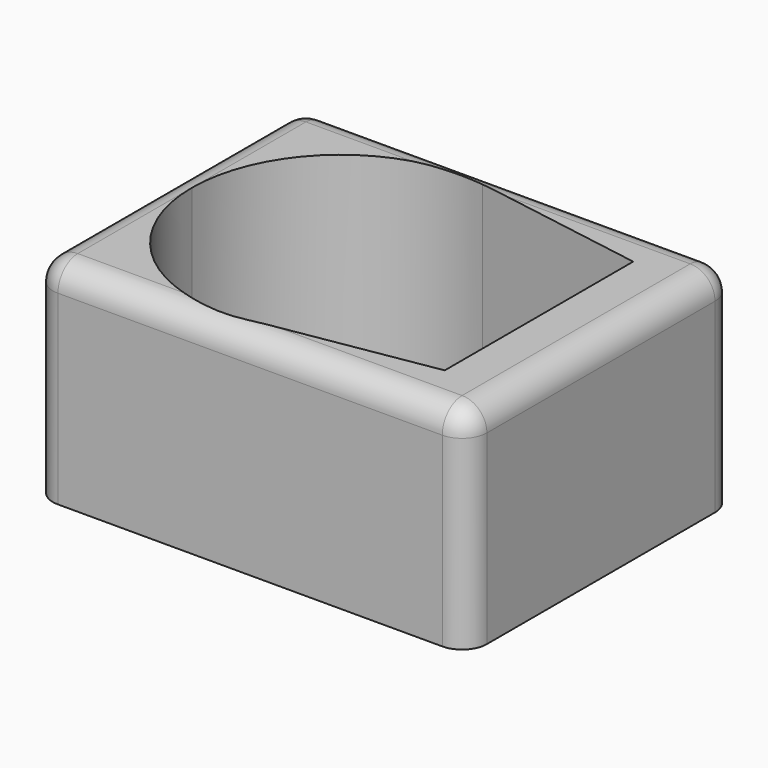
from build123d import *

# Parameters (mm, degrees)
F0_W         = 35
F0_H         = 27
F1_DEPTH     = 15
F2_DEPTH     = 2
F3_T1_DEPTH  = 20
F3_T3_DEPTH  = 23
F3_T5_DEPTH  = 31
F3_S9_W      = 2
F3_S9_H      = 2
F3_T10_DEPTH = 2
F3_S15_W     = 2
F3_S15_H     = 2
F3_T16_DEPTH = 2
F3_S21_W     = 2
F3_S21_H     = 2
F3_T22_DEPTH = 2
F3_S27_W     = 2
F3_S27_H     = 2
F3_T28_DEPTH = 2


# Not quite as in the source:
# - a fillet or chamfer that OpenCascade refuses, or shapes differently, is made with other operations: its cross-section is extruded or revolved along the edge and cut away or added


with BuildPart() as f1:
    # F0 (on Top) → F1 (new body)
    with BuildSketch(Plane.XY):
        with Locations((-13.2022674233, 7.6325895488)):
            Rectangle(F0_W, F0_H)
        with BuildLine():
            Line((-14.73041686, 19.4694728107), (-0.7022674233, 17.1325895488))
            Line((-0.7022674233, 17.1325895488), (-0.7022674233, 7.6325895488))
            Line((-0.7022674233, 7.6325895488), (-0.7022674233, -1.8674104512))
            Line((-0.7022674233, -1.8674104512), (-14.73041686, -4.2042937131))
            ThreePointArc((-14.73041686, -4.2042937131), (-24.4591286842, -1.5233431387), (-28.7022674233, 7.6325895488))
            ThreePointArc((-28.7022674233, 7.6325895488), (-24.4591286842, 16.7885222364), (-14.73041686, 19.4694728107))
        make_face(mode=Mode.SUBTRACT)
    extrude(amount=F1_DEPTH)

    # F0 (on Top) → F2 (join)
    with BuildSketch(Plane.XY):
        with Locations((-13.2022674233, 7.6325895488)):
            Rectangle(F0_W, F0_H)
        with BuildLine():
            Line((-14.73041686, 19.4694728107), (-0.7022674233, 17.1325895488))
            Line((-0.7022674233, 17.1325895488), (-0.7022674233, 7.6325895488))
            Line((-0.7022674233, 7.6325895488), (-0.7022674233, -1.8674104512))
            Line((-0.7022674233, -1.8674104512), (-14.73041686, -4.2042937131))
            ThreePointArc((-14.73041686, -4.2042937131), (-24.4591286842, -1.5233431387), (-28.7022674233, 7.6325895488))
            ThreePointArc((-28.7022674233, 7.6325895488), (-24.4591286842, 16.7885222364), (-14.73041686, 19.4694728107))
        make_face(mode=Mode.SUBTRACT)
        with BuildLine():
            ThreePointArc((-14.73041686, -4.2042937131), (-7.5463347357, -0.1242717121), (-4.7022674233, 7.6325895488))
            Line((-4.7022674233, 7.6325895488), (-28.7022674233, 7.6325895488))
            ThreePointArc((-28.7022674233, 7.6325895488), (-24.4591286842, -1.5233431387), (-14.73041686, -4.2042937131))
        make_face()
        with BuildLine():
            ThreePointArc((-4.7022674233, 7.6325895488), (-7.5463347357, 15.3894508097), (-14.73041686, 19.4694728107))
            ThreePointArc((-14.73041686, 19.4694728107), (-24.4591286842, 16.7885222364), (-28.7022674233, 7.6325895488))
            Line((-28.7022674233, 7.6325895488), (-4.7022674233, 7.6325895488))
        make_face()
        with BuildLine():
            Line((-0.7022674233, 7.6325895488), (-0.7022674233, 17.1325895488))
            Line((-0.7022674233, 17.1325895488), (-14.73041686, 19.4694728107))
            ThreePointArc((-14.73041686, 19.4694728107), (-7.5463347357, 15.3894508097), (-4.7022674233, 7.6325895488))
            Line((-4.7022674233, 7.6325895488), (-0.7022674233, 7.6325895488))
        make_face()
        with BuildLine():
            Line((-0.7022674233, -1.8674104512), (-0.7022674233, 7.6325895488))
            Line((-0.7022674233, 7.6325895488), (-4.7022674233, 7.6325895488))
            ThreePointArc((-4.7022674233, 7.6325895488), (-7.5463347357, -0.1242717121), (-14.73041686, -4.2042937131))
            Line((-14.73041686, -4.2042937131), (-0.7022674233, -1.8674104512))
        make_face()
    extrude(amount=-F2_DEPTH)

    # F3: fillet of radius 2 on 8 edges, made by hand

    # F3_s2 → F3_t1 (cut)
    with BuildSketch(Plane.XY.offset(-7)):
        with BuildLine():
            ThreePointArc((-30.7022674233, -3.8674104512), (-30.1164809856, -5.2816240135), (-28.7022674233, -5.8674104512))
            Line((-28.7022674233, -5.8674104512), (-30.7022674233, -5.8674104512))
            Line((-30.7022674233, -5.8674104512), (-30.7022674233, -3.8674104512))
        make_face()
        with BuildLine():
            ThreePointArc((-30.7022674233, 19.1325895488), (-30.1164809856, 20.5468031112), (-28.7022674233, 21.1325895488))
            Line((-28.7022674233, 21.1325895488), (-30.7022674233, 21.1325895488))
            Line((-30.7022674233, 21.1325895488), (-30.7022674233, 19.1325895488))
        make_face()
        with BuildLine():
            ThreePointArc((4.2977325767, -3.8674104512), (3.7119461391, -5.2816240135), (2.2977325767, -5.8674104512))
            Line((2.2977325767, -5.8674104512), (4.2977325767, -5.8674104512))
            Line((4.2977325767, -5.8674104512), (4.2977325767, -3.8674104512))
        make_face()
        with BuildLine():
            ThreePointArc((4.2977325767, 19.1325895488), (3.7119461391, 20.5468031112), (2.2977325767, 21.1325895488))
            Line((2.2977325767, 21.1325895488), (4.2977325767, 21.1325895488))
            Line((4.2977325767, 21.1325895488), (4.2977325767, 19.1325895488))
        make_face()
    extrude(amount=F3_T1_DEPTH, mode=Mode.SUBTRACT)

    # F3_s4 → F3_t3 (cut)
    with BuildSketch(Plane.XZ.offset(-19.1325895488)):
        with BuildLine():
            ThreePointArc((-30.7022674233, 13), (-30.1164809856, 14.4142135624), (-28.7022674233, 15))
            Line((-28.7022674233, 15), (-30.7022674233, 15))
            Line((-30.7022674233, 15), (-30.7022674233, 13))
        make_face()
        with BuildLine():
            ThreePointArc((4.2977325767, 13), (3.7119461391, 14.4142135624), (2.2977325767, 15))
            Line((2.2977325767, 15), (4.2977325767, 15))
            Line((4.2977325767, 15), (4.2977325767, 13))
        make_face()
    extrude(amount=F3_T3_DEPTH, mode=Mode.SUBTRACT)

    # F3_s6 → F3_t5 (cut)
    with BuildSketch(Plane.YZ.offset(-28.7022674233)):
        with BuildLine():
            ThreePointArc((21.1325895488, 13), (20.5468031112, 14.4142135624), (19.1325895488, 15))
            Line((19.1325895488, 15), (21.1325895488, 15))
            Line((21.1325895488, 15), (21.1325895488, 13))
        make_face()
        with BuildLine():
            ThreePointArc((-3.8674104512, 15), (-5.2816240135, 14.4142135624), (-5.8674104512, 13))
            Line((-5.8674104512, 13), (-5.8674104512, 15))
            Line((-5.8674104512, 15), (-3.8674104512, 15))
        make_face()
    extrude(amount=F3_T5_DEPTH, mode=Mode.SUBTRACT)


with BuildPart() as f3_tool8:
    # F3_s9 → F3_t10 (new body)
    with BuildSketch(Plane.YZ.offset(-28.7022674233)):
        with Locations((-4.8674104512, 14)):
            Rectangle(F3_S9_W, F3_S9_H)
    extrude(amount=-F3_T10_DEPTH)

    # F3_s11 → F3_t12 (revolve, cut)
    with BuildSketch(Plane(origin=(-28.7022674233, -3.8674104512, 13), x_dir=(0, 0.7071067812, -0.7071067812), z_dir=(0, 0.7071067812, 0.7071067812))):
        with BuildLine():
            ThreePointArc((0, -2), (2, 0), (0, 2))
            Line((0, 2), (0, -2))
        make_face()
    revolve(axis=Axis((-28.7022674233, -3.8674104512, 13), (-1, 0, 0)), mode=Mode.SUBTRACT)


with BuildPart() as f1_1:
    add(f1.part)

    # F3_t7: cut F3_tool8
    add(f3_tool8.part, mode=Mode.SUBTRACT)


with BuildPart() as f3_tool14:
    # F3_s15 → F3_t16 (new body)
    with BuildSketch(Plane.YZ.offset(-28.7022674233)):
        with Locations((20.1325895488, 14)):
            Rectangle(F3_S15_W, F3_S15_H)
    extrude(amount=-F3_T16_DEPTH)

    # F3_s17 → F3_t18 (revolve, cut)
    with BuildSketch(Plane(origin=(-28.7022674233, 19.1325895488, 13), x_dir=(0, -0.7071067812, -0.7071067812), z_dir=(0, 0.7071067812, -0.7071067812))):
        with BuildLine():
            ThreePointArc((0, -2), (2, 0), (0, 2))
            Line((0, 2), (0, -2))
        make_face()
    revolve(axis=Axis((-28.7022674233, 19.1325895488, 13), (-1, 0, 0)), mode=Mode.SUBTRACT)


with BuildPart() as f1_2:
    add(f1_1.part)

    # F3_t13: cut F3_tool14
    add(f3_tool14.part, mode=Mode.SUBTRACT)


with BuildPart() as f3_tool20:
    # F3_s21 → F3_t22 (new body)
    with BuildSketch(Plane.YZ.offset(2.2977325767)):
        with Locations((20.1325895488, 14)):
            Rectangle(F3_S21_W, F3_S21_H)
    extrude(amount=F3_T22_DEPTH)

    # F3_s23 → F3_t24 (revolve, cut)
    with BuildSketch(Plane(origin=(2.2977325767, 19.1325895488, 13), x_dir=(0, -0.7071067812, -0.7071067812), z_dir=(0, -0.7071067812, 0.7071067812))):
        with BuildLine():
            ThreePointArc((0, -2), (2, 0), (0, 2))
            Line((0, 2), (0, -2))
        make_face()
    revolve(axis=Axis((2.2977325767, 19.1325895488, 13), (1, 0, 0)), mode=Mode.SUBTRACT)


with BuildPart() as f1_3:
    add(f1_2.part)

    # F3_t19: cut F3_tool20
    add(f3_tool20.part, mode=Mode.SUBTRACT)


with BuildPart() as f3_tool26:
    # F3_s27 → F3_t28 (new body)
    with BuildSketch(Plane.YZ.offset(2.2977325767)):
        with Locations((-4.8674104512, 14)):
            Rectangle(F3_S27_W, F3_S27_H)
    extrude(amount=F3_T28_DEPTH)

    # F3_s29 → F3_t30 (revolve, cut)
    with BuildSketch(Plane(origin=(2.2977325767, -3.8674104512, 13), x_dir=(0, 0.7071067812, -0.7071067812), z_dir=(0, -0.7071067812, -0.7071067812))):
        with BuildLine():
            ThreePointArc((0, -2), (2, 0), (0, 2))
            Line((0, 2), (0, -2))
        make_face()
    revolve(axis=Axis((2.2977325767, -3.8674104512, 13), (1, 0, 0)), mode=Mode.SUBTRACT)


with BuildPart() as f1_4:
    add(f1_3.part)

    # F3_t25: cut F3_tool26
    add(f3_tool26.part, mode=Mode.SUBTRACT)


solid = f1_4.part
